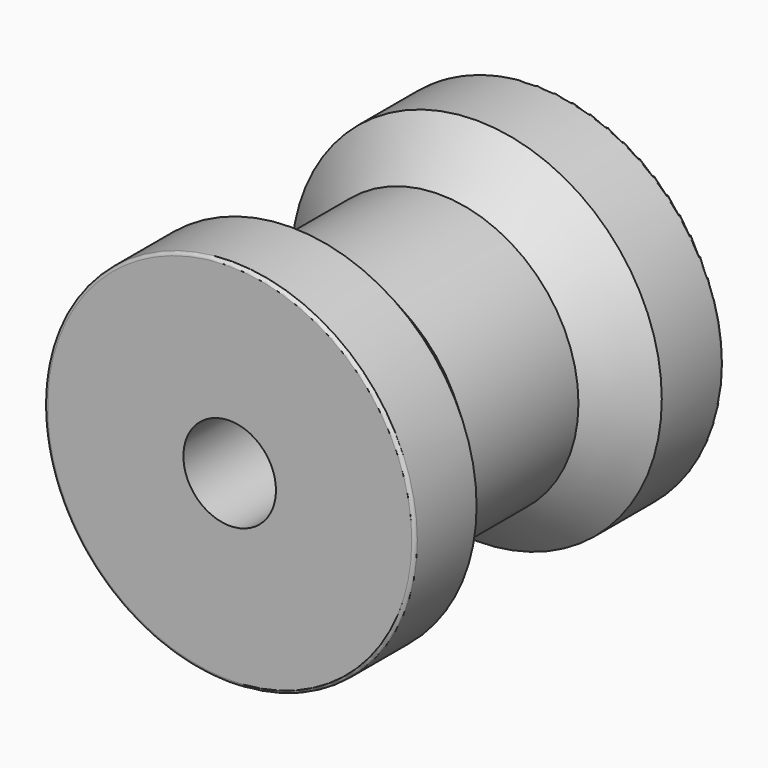
from build123d import *

# Parameters (mm, degrees)
F0_R     = 6
F1_DEPTH = 4
F2_R     = 4.5
F3_DEPTH = 4.5
F4_R     = 6
F4_R_2   = 4.5
F5_DEPTH = 4
F6_R     = 1.5
F7_DEPTH = 15
F8_SIZE  = 1.49999
F9_R     = 0.1


# Not quite as in the source:
# - a fillet or chamfer is up to 0.001 mm smaller than in the source, because OpenCascade refuses the exact size


with BuildPart() as f1:
    # F0 (on Front) → F1 (new body)
    with BuildSketch(Plane.XZ):
        Circle(F0_R)
    extrude(amount=F1_DEPTH)

    # F2 (on face) → F3 (join)
    with BuildSketch(Plane.XZ.offset(4)):
        Circle(F2_R)
    extrude(amount=F3_DEPTH)

    # F4 (on face) → F5 (join)
    with BuildSketch(Plane.XZ.offset(8.5)):
        Circle(F4_R)
        Circle(F4_R_2, mode=Mode.SUBTRACT)
        Circle(F4_R_2)
    extrude(amount=F5_DEPTH)

    # F6 (on face) → F7 (cut)
    with BuildSketch(Plane.XZ.offset(12.5)):
        Circle(F6_R)
    extrude(amount=-F7_DEPTH, mode=Mode.SUBTRACT)

    # F8 (size 1.5 in the source; OpenCascade refuses exactly that, so slightly less here)
    f8_edges = [f1.edges().sort_by_distance(p)[0] for p in [
        (-6, -8.5, 0),
        (-6, -4, 0),
    ]]
    chamfer(f8_edges, length=F8_SIZE)

    # F9
    f9_edges = [f1.edges().sort_by_distance(p)[0] for p in [
        (-6, -12.5, 0),
        (-6, 0, 0),
    ]]
    fillet(f9_edges, radius=F9_R)


solid = f1.part
